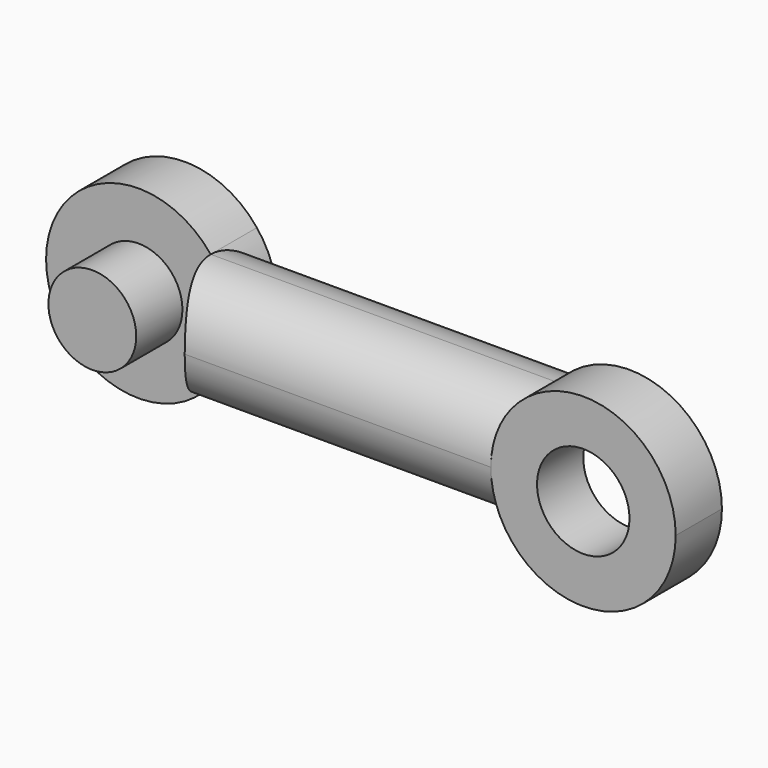
from build123d import *

# Parameters (mm, degrees)
F1_DEPTH = 6.35
F2_R     = 6.3499
F0_R     = 5.08
F3_DEPTH = 6.35
F0_R_2   = 4.826
F4_DEPTH = 6.35
F5_DEPTH = 6.35


# Not quite as in the source:
# - a fillet or chamfer is up to 0.001 mm smaller than in the source, because OpenCascade refuses the exact size


with BuildPart() as f1:
    # F0 (on Front) → F1 (new body, symmetric)
    with BuildSketch(Plane.XZ):
        with BuildLine():
            Line((19.05, 6.35), (-19.05, 6.35))
            ThreePointArc((-19.05, 6.35), (-17.3945407024, 3.3649028089), (-16.821147458, 0))
            ThreePointArc((-16.821147458, 0), (-17.3945407024, -3.3649028089), (-19.05, -6.35))
            Line((-19.05, -6.35), (19.05, -6.35))
            ThreePointArc((19.05, -6.35), (16.821147458, 0), (19.05, 6.35))
        make_face()
    extrude(amount=F1_DEPTH, both=True)

    # F2 (radius 6.35 in the source; OpenCascade refuses exactly that, so slightly less here)
    f2_edges = [f1.edges().sort_by_distance(p)[0] for p in [
        (0, -6.35, 6.35),
        (0, 6.35, 6.35),
        (0, -6.35, -6.35),
        (0, 6.35, -6.35),
    ]]
    fillet(f2_edges, radius=F2_R)

    # F0 (on Front) → F3 (join)
    with BuildSketch(Plane.XZ):
        with BuildLine():
            ThreePointArc((37.141147458, 0), (30.3460502669, 9.5866067556), (19.05, 6.35))
            Line((19.05, 6.35), (19.05, -6.35))
            ThreePointArc((19.05, -6.35), (30.3460502669, -9.5866067556), (37.141147458, 0))
        make_face()
        with Locations((26.981147458, 0)):
            Circle(F0_R, mode=Mode.SUBTRACT)
        with BuildLine():
            Line((19.05, -6.35), (19.05, 6.35))
            ThreePointArc((19.05, 6.35), (16.821147458, 0), (19.05, -6.35))
        make_face()
    extrude(amount=F3_DEPTH)

    # F0 (on Front) → F4 (join)
    with BuildSketch(Plane.XZ):
        with BuildLine():
            Line((-19.05, -6.35), (-19.05, 6.35))
            ThreePointArc((-19.05, 6.35), (-37.141147458, 0), (-19.05, -6.35))
        make_face()
        with Locations((-26.981147458, 0)):
            Circle(F0_R_2, mode=Mode.SUBTRACT)
        with BuildLine():
            ThreePointArc((-16.821147458, 0), (-17.3945407024, 3.3649028089), (-19.05, 6.35))
            Line((-19.05, 6.35), (-19.05, -6.35))
            ThreePointArc((-19.05, -6.35), (-17.3945407024, -3.3649028089), (-16.821147458, 0))
        make_face()
    extrude(amount=-F4_DEPTH)

    # F0 (on Front) → F5 (join, symmetric)
    with BuildSketch(Plane.XZ):
        with Locations((-26.981147458, 0)):
            Circle(F0_R_2)
    extrude(amount=F5_DEPTH, both=True)


solid = f1.part
